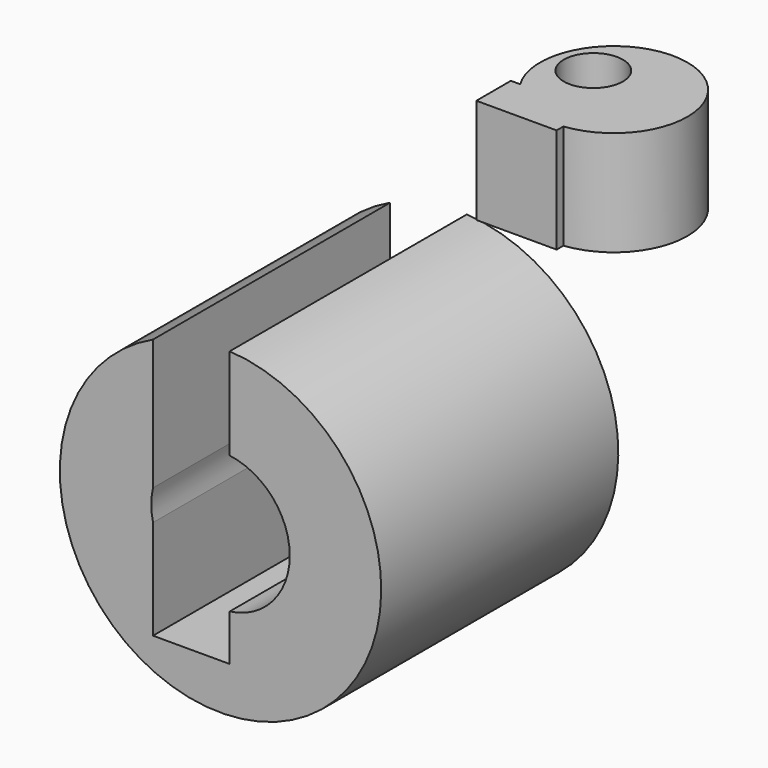
from build123d import *

# Parameters (mm, degrees)
F1_DEPTH = 90.678
F2_R     = 25.5758086302
F3_DEPTH = 141.732
F5_DEPTH = 256.032


# Not quite as in the source:
# - the program builds the solid bodies; features that only make, move or delete a surface that nothing else refers to are left out


with BuildPart() as f1:
    # F0 (on Top) → F1 (new body)
    with BuildSketch(Plane.XY):
        with BuildLine():
            Line((-30.178046057, 12.7954334021), (-38.2321402431, 12.7954334021))
            Line((-38.2321402431, 12.7954334021), (-38.2321402431, -24.5117340237))
            Line((-38.2321402431, -24.5117340237), (31.1406925321, -24.5117340237))
            Line((31.1406925321, -24.5117340237), (31.1406925321, -17.1442935736))
            ThreePointArc((31.1406925321, -17.1442935736), (-3.8710651375, -11.08843806), (-30.178046057, 12.7954334021))
        make_face()
        with BuildLine():
            ThreePointArc((87.6843044367, 46.0943952203), (6.7480431649, 107.3323624507), (-30.178046057, 12.7954334021))
            Line((-30.178046057, 12.7954334021), (31.1406925321, 12.7954334021))
            Line((31.1406925321, 12.7954334021), (31.1406925321, -17.1442935736))
            ThreePointArc((31.1406925321, -17.1442935736), (71.4870223798, 3.6788561821), (87.6843044367, 46.0943952203))
        make_face()
        with BuildLine():
            Line((31.1406925321, 12.7954334021), (-30.178046057, 12.7954334021))
            ThreePointArc((-30.178046057, 12.7954334021), (-3.8710651375, -11.08843806), (31.1406925321, -17.1442935736))
            Line((31.1406925321, -17.1442935736), (31.1406925321, 12.7954334021))
        make_face()
    extrude(amount=F1_DEPTH)

    # F2 (on face) → F3 (cut)
    with BuildSketch(Plane.XY.offset(90.678)):
        with Locations((-4.1088564321, 59.2082738876)):
            Circle(F2_R)
    extrude(amount=-F3_DEPTH, mode=Mode.SUBTRACT)


with BuildPart() as f5:
    # F4 (on Front) → F5 (new body)
    with BuildSketch(Plane.XZ):
        with BuildLine():
            ThreePointArc((64.8145101963, -153.4280627966), (26.9208728789, -58.1070194145), (-66.0748556256, -14.819335941))
            Line((-66.0748556256, -14.819335941), (-66.0748556256, -94.1540102087))
            ThreePointArc((-66.0748556256, -94.1540102087), (-29.0116634578, -114.0497511318), (-14.2174317784, -153.4280627966))
            ThreePointArc((-14.2174317784, -153.4280627966), (-29.0116634578, -192.8063744613), (-66.0748556256, -212.7021153845))
            Line((-66.0748556256, -212.7021153845), (-66.0748556256, -252.6962310076))
            Line((-66.0748556256, -252.6962310076), (-132.3496177793, -252.6962310076))
            Line((-132.3496177793, -252.6962310076), (-132.3496177793, -166.6355990123))
            ThreePointArc((-132.3496177793, -166.6355990123), (-133.8262603336, -153.4280627966), (-132.3496177793, -140.2205265809))
            Line((-132.3496177793, -140.2205265809), (-132.3496177793, -27.4383613793))
            ThreePointArc((-132.3496177793, -27.4383613793), (-148.7798507212, -270.4185519652), (64.8145101963, -153.4280627966))
        make_face()
    extrude(amount=F5_DEPTH)


solid = Compound([f1.part, f5.part])
